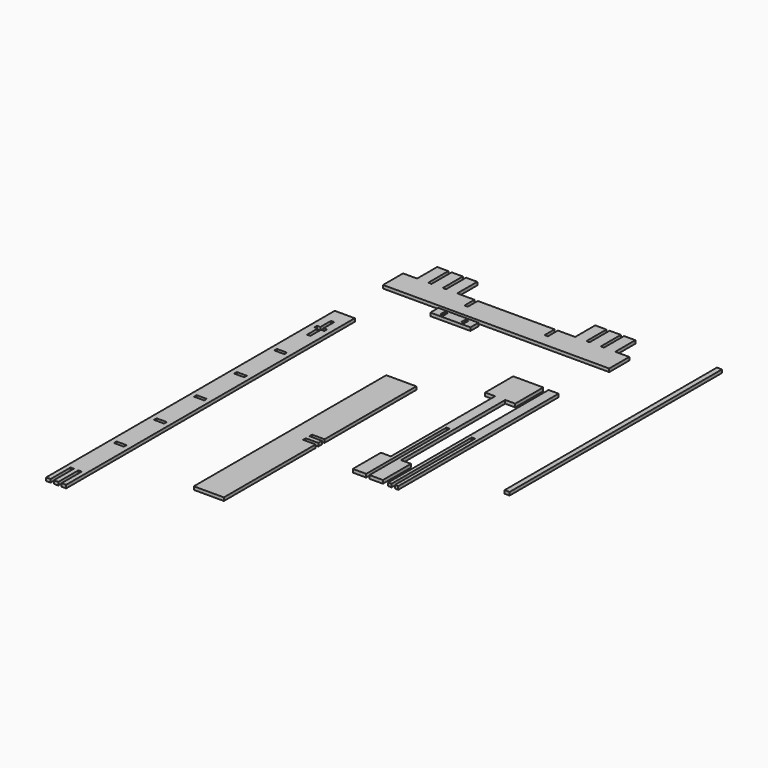
from build123d import *

# Parameters (mm, degrees)
F2_DEPTH = 16
F1_W     = 200
F1_H     = 50
F1_W_2   = 16.6
F1_H_2   = 25
F1_W_3   = 16
F1_W_4   = 50
F1_H_3   = 16.6
F3_DEPTH = 16.6
F1_W_5   = 25
F1_H_4   = 1324
F4_DEPTH = 16


# Not quite as in the source:
# - a feature names something its author has since deleted; it is built from what else it names


with BuildPart() as f2:
    # F1 (on Top) → F2 (new body)
    with BuildSketch(Plane.XY):
        Polygon((1826.8150956472, 2554.895401001), (1826.8150956472, 2429.895401001), (2955.2150956472, 2429.895401001), (2955.2150956472, 2554.895401001), (2885.2150956472, 2554.895401001), (2885.2150956472, 2679.895401001), (2829.2150956472, 2679.895401001), (2829.2150956472, 2554.895401001), (2813.2150956472, 2554.895401001), (2813.2150956472, 2679.895401001), (2757.2150956472, 2679.895401001), (2757.2150956472, 2554.895401001), (2741.2150956472, 2554.895401001), (2741.2150956472, 2679.895401001), (2685.2150956472, 2679.895401001), (2685.2150956472, 2554.895401001), (2599.1797067006, 2554.895401001), (2599.1797067006, 2492.395401001), (2582.5797067006, 2492.395401001), (2582.5797067006, 2554.895401001), (2199.4504845937, 2554.895401001), (2199.4504845937, 2492.395401001), (2182.8504845937, 2492.395401001), (2182.8504845937, 2554.895401001), (2096.8150956472, 2554.895401001), (2096.8150956472, 2679.895401001), (2041.2150956472, 2679.895401001), (2041.2150956472, 2554.895401001), (2024.6150956472, 2554.895401001), (2024.6150956472, 2679.895401001), (1969.0150956472, 2679.895401001), (1969.0150956472, 2554.895401001), (1952.4150956472, 2554.895401001), (1952.4150956472, 2679.895401001), (1896.8150956472, 2679.895401001), (1896.8150956472, 2554.895401001), align=None)
    extrude(amount=F2_DEPTH)


with BuildPart() as f2b:
    # F1 (on Top) → F2, piece 2 (new body)
    with BuildSketch(Plane.XY):
        with Locations((2216.0817146301, 2388.1756305695)):
            Rectangle(F1_W, F1_H)
        with Locations((2163.7817146301, 2388.1756305695)):
            Rectangle(F1_W_2, F1_H_2, mode=Mode.SUBTRACT)
        with Locations((2268.0817146301, 2388.1756305695)):
            Rectangle(F1_W_3, F1_H_2, mode=Mode.SUBTRACT)
    extrude(amount=F2_DEPTH)


with BuildPart() as f2c:
    # F1 (on Top) → F2, piece 3 (new body)
    with BuildSketch(Plane.XY):
        Polygon((2917.0303050995, 1140.9330368042), (2933.7303050995, 1140.9330368042), (2933.7303050995, 2140.9330368042), (2883.7303050995, 2140.9330368042), (2883.7303050995, 1140.9330368042), (2900.4303050995, 1140.9330368042), (2900.4303050995, 1640.9330368042), (2917.0303050995, 1640.9330368042), align=None)
    extrude(amount=F2_DEPTH)


with BuildPart() as f2d:
    # F1 (on Top) → F2, piece 4 (new body)
    with BuildSketch(Plane.XY):
        Polygon((1916.0817667643, 2142.0231616099), (1816.0817667643, 2142.0231616099), (1816.0817667643, 342.0231616099), (1838.348433431, 342.0231616099), (1838.348433431, 467.0231616099), (1854.948433431, 467.0231616099), (1854.948433431, 342.0231616099), (1877.2151000977, 342.0231616099), (1877.2151000977, 467.0231616099), (1893.8151000977, 467.0231616099), (1893.8151000977, 342.0231616099), (1916.0817667643, 342.0231616099), align=None)
        with Locations((1866.0817667643, 742.0231616099)):
            Rectangle(F1_W_4, F1_H_3, mode=Mode.SUBTRACT)
        with Locations((1866.0817667643, 992.0231616099)):
            Rectangle(F1_W_4, F1_H_3, mode=Mode.SUBTRACT)
        with Locations((1866.0817667643, 1242.0231616099)):
            Rectangle(F1_W_4, F1_H_3, mode=Mode.SUBTRACT)
        with Locations((1866.0817667643, 1492.0231616099)):
            Rectangle(F1_W_4, F1_H_3, mode=Mode.SUBTRACT)
        with Locations((1866.0817667643, 1742.0231616099)):
            Rectangle(F1_W_4, F1_H_3, mode=Mode.SUBTRACT)
        Polygon((1874.3817667643, 2000.3231616099), (1891.0817667643, 2000.3231616099), (1891.0817667643, 1983.7231616099), (1874.3817667643, 1983.7231616099), (1874.3817667643, 1917.0231616099), (1857.7817667643, 1917.0231616099), (1857.7817667643, 1983.7231616099), (1841.0817667643, 1983.7231616099), (1841.0817667643, 2000.3231616099), (1857.7817667643, 2000.3231616099), (1857.7817667643, 2067.0231616099), (1874.3817667643, 2067.0231616099), align=None, mode=Mode.SUBTRACT)
    extrude(amount=F2_DEPTH)


with BuildPart() as f2e:
    # F1 (on Top) → F2, piece 5 (new body)
    with BuildSketch(Plane.XY):
        Polygon((2312.2333049774, 1843.0356502533), (2312.2333049774, 643.0356502533), (2462.2333049774, 643.0356502533), (2462.2333049774, 1215.0856502533), (2399.7333049774, 1215.0856502533), (2399.7333049774, 1231.6856502533), (2462.2333049774, 1231.6856502533), (2462.2333049774, 1254.3856502533), (2399.7333049774, 1254.3856502533), (2399.7333049774, 1270.9856502533), (2462.2333049774, 1270.9856502533), (2462.2333049774, 1843.0356502533), align=None)
    extrude(amount=F2_DEPTH)


with BuildPart() as f3:
    # F1 (on Top) → F3 (new body)
    with BuildSketch(Plane.XY):
        Polygon((2855.0214290619, 1968.6681032181), (2855.0214290619, 2143.6681032181), (2705.0214290619, 2143.6681032181), (2705.0214290619, 1968.6681032181), (2754.7214290619, 1968.6681032181), (2754.7214290619, 1318.6681032181), (2705.0214290619, 1318.6681032181), (2705.0214290619, 1143.6681032181), (2771.7214290619, 1143.6681032181), (2771.7214290619, 1643.6681032181), (2788.3214290619, 1643.6681032181), (2788.3214290619, 1143.6681032181), (2855.0214290619, 1143.6681032181), (2855.0214290619, 1318.6681032181), (2805.3214290619, 1318.6681032181), (2805.3214290619, 1968.6681032181), align=None)
    extrude(amount=F3_DEPTH)


with BuildPart() as f4:
    # F1 (on Top) → F4 (new body)
    with BuildSketch(Plane.XY):
        with Locations((3290.2781486511, 2036.1644620895)):
            Rectangle(F1_W_5, F1_H_4)
    extrude(amount=F4_DEPTH)


solid = Compound([f2.part, f2b.part, f2c.part, f2d.part, f2e.part, f3.part, f4.part])
